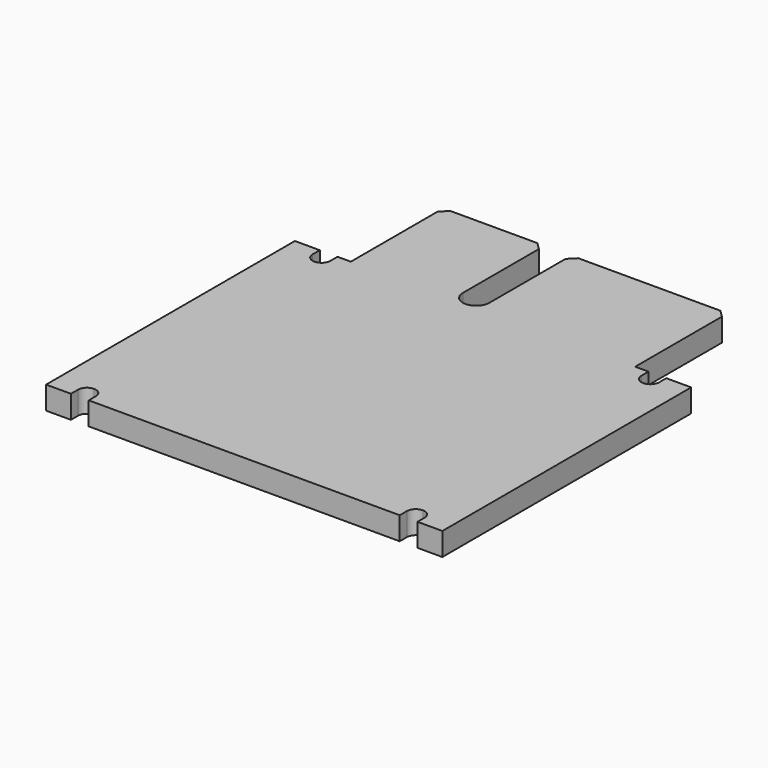
from build123d import *

# Parameters (mm, degrees)
F0_W     = 28.321
F0_H     = 30.48
F1_DEPTH = 1.64
F2_W     = 1.905
F2_H     = 8.255
F2_W_2   = 1.27
F2_H_2   = 1.27
F3_DEPTH = 25
F4_R     = 0.95249
F5_SIZE  = 0.507
F6_R     = 0.63499


# Not quite as in the source:
# - a fillet or chamfer is up to 0.001 mm smaller than in the source, because OpenCascade refuses the exact size


with BuildPart() as f1:
    # F0 (on Top) → F1 (new body)
    with BuildSketch(Plane.XY):
        with Locations((0, -15.24)):
            Rectangle(F0_W, F0_H)
    extrude(amount=F1_DEPTH)

    # F2 (on Top) → F3 (cut)
    with BuildSketch(Plane.XY):
        Polygon((-10.16, 0), (-14.1605, 0), (-14.1605, -8.255), (-12.3825, -8.255), (-12.3825, -9.525), (-11.1125, -9.525), (-11.1125, -8.255), (-10.16, -8.255), align=None)
        with Locations((-1.9685, -4.1275)):
            Rectangle(F2_W, F2_H)
        Polygon((14.1605, -8.255), (14.1605, 0), (10.16, 0), (10.16, -8.255), (11.1125, -8.255), (11.1125, -9.525), (12.3825, -9.525), (12.3825, -8.255), align=None)
        with Locations((-11.7475, -29.845)):
            Rectangle(F2_W_2, F2_H_2)
        with Locations((11.7475, -29.845)):
            Rectangle(F2_W_2, F2_H_2)
    extrude(amount=F3_DEPTH, mode=Mode.SUBTRACT)

    # F4 (radius 0.9525 in the source; OpenCascade refuses exactly that, so slightly less here)
    f4_edges = [f1.edges().sort_by_distance(p)[0] for p in [
        (-2.921, -8.255, 0.82),
        (-1.016, -8.255, 0.82),
    ]]
    fillet(f4_edges, radius=F4_R)

    # F5
    f5_edges = [f1.edges().sort_by_distance(p)[0] for p in [
        (10.16, 0, 0.82),
        (-1.016, 0, 0.82),
        (-2.921, 0, 0.82),
        (-10.16, 0, 0.82),
    ]]
    chamfer(f5_edges, length=F5_SIZE)

    # F6 (radius 0.635 in the source; OpenCascade refuses exactly that, so slightly less here)
    f6_edges = [f1.edges().sort_by_distance(p)[0] for p in [
        (12.3825, -29.21, 0.82),
        (-12.3825, -29.21, 0.82),
        (-11.1125, -29.21, 0.82),
        (11.1125, -29.21, 0.82),
        (11.1125, -9.525, 0.82),
        (12.3825, -9.525, 0.82),
        (-12.3825, -9.525, 0.82),
        (-11.1125, -9.525, 0.82),
    ]]
    fillet(f6_edges, radius=F6_R)


solid = f1.part
